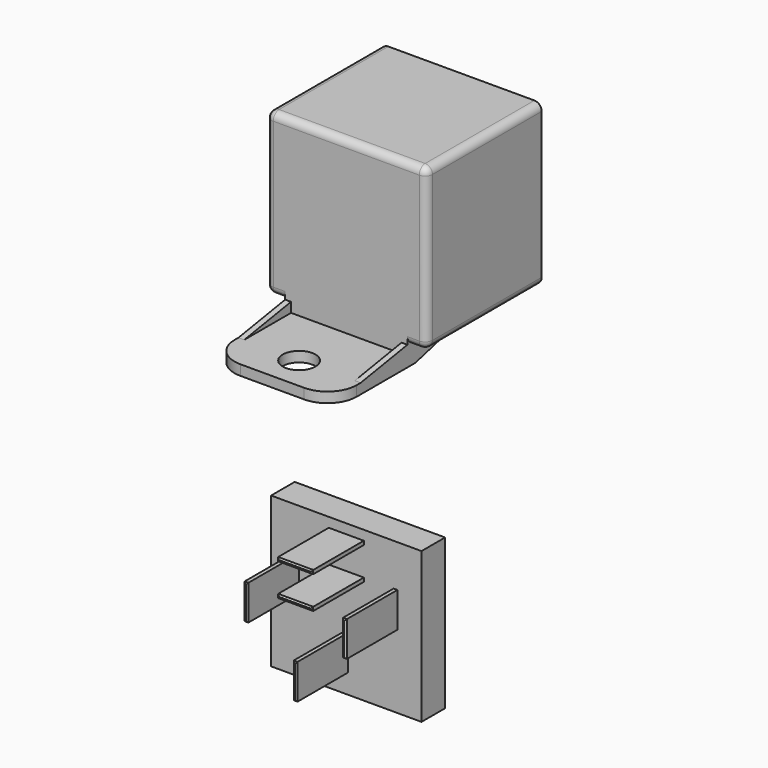
from build123d import *

# Parameters (mm, degrees)
F0_W          = 26.162
F0_H          = 26.162
F0_W_2        = 0.6604
F0_H_2        = 6.096
F0_W_3        = 6.096
F0_H_3        = 0.6604
F1_DEPTH      = 5.1308
F2_DEPTH      = 11.2522
F3_SIZE       = 0.254
F4_W          = 27.94
F4_H          = 27.94
F4_W_2        = 26.162
F4_H_2        = 26.162
F5_DEPTH      = 25.019
F6_START      = -2.54
F6_DEPTH      = 25.4
F8_DEPTH      = 10.6299
F9_DEPTH      = 9.6139
F10_R         = 2.8448
F11_DEPTH     = 1.778
F12_R         = 5.08
F13_T1_DEPTH  = 25.4
F13_T3_DEPTH  = 26.924
F13_T5_DEPTH  = 25.4
F13_T7_DEPTH  = 2.0701
F13_T9_DEPTH  = 2.0701
F13_S13_W     = 1.2954
F13_S13_H     = 1.2954
F13_T14_DEPTH = 1.2954
F13_S19_W     = 1.2954
F13_S19_H     = 1.2954
F13_T20_DEPTH = 1.2954
F13_S25_W     = 1.2954
F13_S25_H     = 1.2954
F13_T26_DEPTH = 1.2954
F13_S31_W     = 1.2954
F13_S31_H     = 1.2954
F13_T32_DEPTH = 1.2954


# Not quite as in the source:
# - a fillet or chamfer that OpenCascade refuses, or shapes differently, is made with other operations: its cross-section is extruded or revolved along the edge and cut away or added


with BuildPart() as f1:
    # F0 (on Front) → F1 (new body)
    with BuildSketch(Plane.XZ):
        Rectangle(F0_W, F0_H)
        with Locations((0, -6.604)):
            Rectangle(F0_W_2, F0_H_2, mode=Mode.SUBTRACT)
        with Locations((-8.5598, 2.7178)):
            Rectangle(F0_W_2, F0_H_2, mode=Mode.SUBTRACT)
        with Locations((0, 5.4356)):
            Rectangle(F0_W_3, F0_H_3, mode=Mode.SUBTRACT)
        with Locations((8.5598, 2.7178)):
            Rectangle(F0_W_2, F0_H_2, mode=Mode.SUBTRACT)
        with Locations((0, 11.0744)):
            Rectangle(F0_W_3, F0_H_3, mode=Mode.SUBTRACT)
        with Locations((0, 11.0744)):
            Rectangle(F0_W_3, F0_H_3)
        with Locations((0, 5.4356)):
            Rectangle(F0_W_3, F0_H_3)
        with Locations((-8.5598, 2.7178)):
            Rectangle(F0_W_2, F0_H_2)
        with Locations((8.5598, 2.7178)):
            Rectangle(F0_W_2, F0_H_2)
        with Locations((0, -6.604)):
            Rectangle(F0_W_2, F0_H_2)
    extrude(amount=-F1_DEPTH)

    # F0 (on Front) → F2 (join)
    with BuildSketch(Plane.XZ):
        with Locations((0, 11.0744)):
            Rectangle(F0_W_3, F0_H_3)
        with Locations((0, 5.4356)):
            Rectangle(F0_W_3, F0_H_3)
        with Locations((-8.5598, 2.7178)):
            Rectangle(F0_W_2, F0_H_2)
        with Locations((8.5598, 2.7178)):
            Rectangle(F0_W_2, F0_H_2)
        with Locations((0, -6.604)):
            Rectangle(F0_W_2, F0_H_2)
    extrude(amount=F2_DEPTH)

    # F3
    f3_edges = [f1.edges().sort_by_distance(p)[0] for p in [
        (0, -11.2522, 5.7658),
        (0, -11.2522, 5.1054),
        (-3.048, -11.2522, 5.4356),
        (3.048, -11.2522, 5.4356),
        (0, -11.2522, 11.4046),
        (0, -11.2522, 10.7442),
        (-3.048, -11.2522, 11.0744),
        (3.048, -11.2522, 11.0744),
        (8.5598, -11.2522, 5.7658),
        (8.89, -11.2522, 2.7178),
        (8.2296, -11.2522, 2.7178),
        (8.5598, -11.2522, -0.3302),
        (-8.5598, -11.2522, 5.7658),
        (-8.2296, -11.2522, 2.7178),
        (-8.89, -11.2522, 2.7178),
        (-8.5598, -11.2522, -0.3302),
        (0, -11.2522, -3.556),
        (0.3302, -11.2522, -6.604),
        (-0.3302, -11.2522, -6.604),
        (0, -11.2522, -9.652),
    ]]
    chamfer(f3_edges, length=F3_SIZE)


with BuildPart() as f5:
    # F4 (on Front) → F5 (new body)
    with BuildSketch(Plane.XZ):
        with Locations((0, 57.826566013)):
            Rectangle(F4_W, F4_H)
        with Locations((0, 57.826566013)):
            Rectangle(F4_W_2, F4_H_2, mode=Mode.SUBTRACT)
        with Locations((0, 57.826566013)):
            Rectangle(F4_W_2, F4_H_2)
    extrude(amount=-F5_DEPTH)

    # F4 (on Front) → F6 (cut)
    with BuildSketch(Plane.XZ.offset(F6_START)):
        with Locations((0, 57.826566013)):
            Rectangle(F4_W_2, F4_H_2)
    extrude(amount=-F6_DEPTH, mode=Mode.SUBTRACT)

    # F7 (on Right) → F8 (join, symmetric)
    with BuildSketch(Plane.YZ):
        Polygon((-16.1036, 40.402166013), (1.7117746174, 40.402166013), (15.24, 43.8772775233), (0, 43.8772775233), (0, 42.180166013), (-10.16, 42.180166013), (-16.1036, 42.180166013), align=None)
        Polygon((0, 42.180166013), (0, 43.8772775233), (-10.16, 42.180166013), align=None)
    extrude(amount=F8_DEPTH, both=True)

    # F7 (on Right) → F9 (cut, symmetric)
    with BuildSketch(Plane.YZ):
        Polygon((0, 42.180166013), (0, 43.8772775233), (-10.16, 42.180166013), align=None)
    extrude(amount=F9_DEPTH, both=True, mode=Mode.SUBTRACT)

    # F10 (on face) → F11 (cut, through all)
    with BuildSketch(Plane(origin=(0, 0, 40.402166013), x_dir=(1, 0, 0), z_dir=(0, 0, -1))):
        with Locations((0, 10.2616)):
            Circle(F10_R)
    extrude(amount=-F11_DEPTH, mode=Mode.SUBTRACT)

    # F12
    f12_edges = [f5.edges().sort_by_distance(p)[0] for p in [
        (-10.6299, -16.1036, 41.291166),
        (10.6299, -16.1036, 41.291166),
    ]]
    fillet(f12_edges, radius=F12_R)

    # F13: fillet of radius 1.27 on 9 edges, made by hand

    # F13_s2 → F13_t1 (cut)
    with BuildSketch(Plane.XY.offset(45.126566013)):
        with BuildLine():
            ThreePointArc((12.7, 0), (13.5980256121, 0.3719743879), (13.97, 1.27))
            Line((13.97, 1.27), (13.97, 0))
            Line((13.97, 0), (12.7, 0))
        make_face()
        with BuildLine():
            ThreePointArc((-12.7, 0), (-13.5980256121, 0.3719743879), (-13.97, 1.27))
            Line((-13.97, 1.27), (-13.97, 0))
            Line((-13.97, 0), (-12.7, 0))
        make_face()
    extrude(amount=F13_T1_DEPTH, mode=Mode.SUBTRACT)

    # F13_s4 → F13_t3 (cut)
    with BuildSketch(Plane.XZ.offset(-28.194)):
        with BuildLine():
            ThreePointArc((13.97, 70.526566013), (13.5980256121, 71.4245916251), (12.7, 71.796566013))
            Line((12.7, 71.796566013), (13.97, 71.796566013))
            Line((13.97, 71.796566013), (13.97, 70.526566013))
        make_face()
        with BuildLine():
            ThreePointArc((-13.97, 70.526566013), (-13.5980256121, 71.4245916251), (-12.7, 71.796566013))
            Line((-12.7, 71.796566013), (-13.97, 71.796566013))
            Line((-13.97, 71.796566013), (-13.97, 70.526566013))
        make_face()
        with BuildLine():
            ThreePointArc((-12.7, 43.856566013), (-13.5980256121, 44.2285404009), (-13.97, 45.126566013))
            Line((-13.97, 45.126566013), (-13.97, 43.856566013))
            Line((-13.97, 43.856566013), (-12.7, 43.856566013))
        make_face()
        with BuildLine():
            ThreePointArc((12.7, 43.856566013), (13.5980256121, 44.2285404009), (13.97, 45.126566013))
            Line((13.97, 45.126566013), (13.97, 43.856566013))
            Line((13.97, 43.856566013), (12.7, 43.856566013))
        make_face()
    extrude(amount=F13_T3_DEPTH, mode=Mode.SUBTRACT)

    # F13_s6 → F13_t5 (cut)
    with BuildSketch(Plane.YZ.offset(-12.7)):
        with BuildLine():
            ThreePointArc((0, 70.526566013), (0.3719743879, 71.4245916251), (1.27, 71.796566013))
            Line((1.27, 71.796566013), (0, 71.796566013))
            Line((0, 71.796566013), (0, 70.526566013))
        make_face()
    extrude(amount=F13_T5_DEPTH, mode=Mode.SUBTRACT)

    # F13_s8 → F13_t7 (cut)
    with BuildSketch(Plane.YZ.offset(-12.7)):
        with BuildLine():
            ThreePointArc((1.27, 43.856566013), (0.3719743879, 44.2285404009), (0, 45.126566013))
            Line((0, 45.126566013), (0, 43.856566013))
            Line((0, 43.856566013), (1.27, 43.856566013))
        make_face()
    extrude(amount=F13_T7_DEPTH, mode=Mode.SUBTRACT)

    # F13_s10 → F13_t9 (cut)
    with BuildSketch(Plane.YZ.offset(10.6299)):
        with BuildLine():
            ThreePointArc((1.27, 43.856566013), (0.3719743879, 44.2285404009), (0, 45.126566013))
            Line((0, 45.126566013), (0, 43.856566013))
            Line((0, 43.856566013), (1.27, 43.856566013))
        make_face()
    extrude(amount=F13_T9_DEPTH, mode=Mode.SUBTRACT)


with BuildPart() as f13_tool12:
    # F13_s13 → F13_t14 (new body)
    with BuildSketch(Plane.YZ.offset(12.7)):
        with Locations((0.6223, 44.478866013)):
            Rectangle(F13_S13_W, F13_S13_H)
    extrude(amount=F13_T14_DEPTH)

    # F13_s15 → F13_t16 (revolve, cut)
    with BuildSketch(Plane(origin=(12.7, 1.27, 45.126566013), x_dir=(0, 0.7071067812, 0.7071067812), z_dir=(0, 0.7071067812, -0.7071067812))):
        with BuildLine():
            ThreePointArc((0, -1.27), (1.27, 0), (0, 1.27))
            Line((0, 1.27), (0, -1.27))
        make_face()
    revolve(axis=Axis((12.7, 1.27, 45.126566013), (1, 0, 0)), mode=Mode.SUBTRACT)


with BuildPart() as f5_1:
    add(f5.part)

    # F13_t11: cut F13_tool12
    add(f13_tool12.part, mode=Mode.SUBTRACT)


with BuildPart() as f13_tool18:
    # F13_s19 → F13_t20 (new body)
    with BuildSketch(Plane.XY.offset(70.526566013)):
        with Locations((13.3477, 0.6223)):
            Rectangle(F13_S19_W, F13_S19_H)
    extrude(amount=F13_T20_DEPTH)

    # F13_s21 → F13_t22 (revolve, cut)
    with BuildSketch(Plane(origin=(12.7, 1.27, 70.526566013), x_dir=(-0.7071067812, 0.7071067812, 0), z_dir=(0.7071067812, 0.7071067812, 0))):
        with BuildLine():
            ThreePointArc((0, -1.27), (1.27, 0), (0, 1.27))
            Line((0, 1.27), (0, -1.27))
        make_face()
    revolve(axis=Axis((12.7, 1.27, 70.526566013), (0, 0, 1)), mode=Mode.SUBTRACT)


with BuildPart() as f5_2:
    add(f5_1.part)

    # F13_t17: cut F13_tool18
    add(f13_tool18.part, mode=Mode.SUBTRACT)


with BuildPart() as f13_tool24:
    # F13_s25 → F13_t26 (new body)
    with BuildSketch(Plane.YZ.offset(-12.7)):
        with Locations((0.6223, 71.174266013)):
            Rectangle(F13_S25_W, F13_S25_H)
    extrude(amount=-F13_T26_DEPTH)

    # F13_s27 → F13_t28 (revolve, cut)
    with BuildSketch(Plane(origin=(-12.7, 1.27, 70.526566013), x_dir=(0, 0.7071067812, -0.7071067812), z_dir=(0, 0.7071067812, 0.7071067812))):
        with BuildLine():
            ThreePointArc((0, -1.27), (1.27, 0), (0, 1.27))
            Line((0, 1.27), (0, -1.27))
        make_face()
    revolve(axis=Axis((-12.7, 1.27, 70.526566013), (-1, 0, 0)), mode=Mode.SUBTRACT)


with BuildPart() as f5_3:
    add(f5_2.part)

    # F13_t23: cut F13_tool24
    add(f13_tool24.part, mode=Mode.SUBTRACT)


with BuildPart() as f13_tool30:
    # F13_s31 → F13_t32 (new body)
    with BuildSketch(Plane.YZ.offset(-12.7)):
        with Locations((0.6223, 44.478866013)):
            Rectangle(F13_S31_W, F13_S31_H)
    extrude(amount=-F13_T32_DEPTH)

    # F13_s33 → F13_t34 (revolve, cut)
    with BuildSketch(Plane(origin=(-12.7, 1.27, 45.126566013), x_dir=(0, 0.7071067812, 0.7071067812), z_dir=(0, -0.7071067812, 0.7071067812))):
        with BuildLine():
            ThreePointArc((0, -1.27), (1.27, 0), (0, 1.27))
            Line((0, 1.27), (0, -1.27))
        make_face()
    revolve(axis=Axis((-12.7, 1.27, 45.126566013), (-1, 0, 0)), mode=Mode.SUBTRACT)


with BuildPart() as f5_4:
    add(f5_3.part)

    # F13_t29: cut F13_tool30
    add(f13_tool30.part, mode=Mode.SUBTRACT)


solid = Compound([f1.part, f5_4.part])
